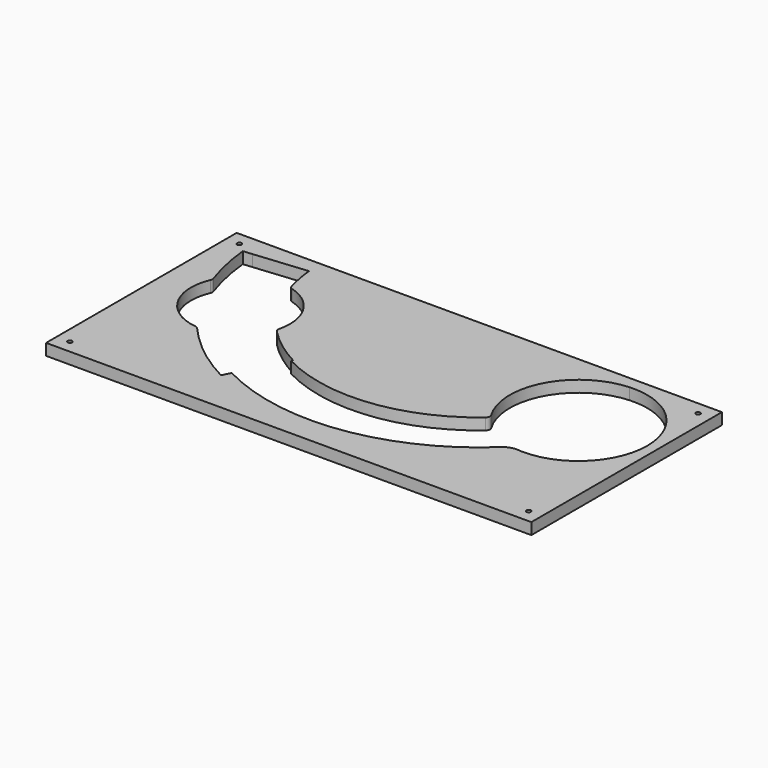
from build123d import *

# Parameters (mm, degrees)
F0_W     = 550
F0_H     = 270
F1_DEPTH = 13
F2_R     = 2.5
F3_DEPTH = 25
F4_R     = 5
F5_R     = 20


with BuildPart() as f1:
    # F0 (on Top) → F1 (new body)
    with BuildSketch(Plane.XY):
        with Locations((275, -135)):
            Rectangle(F0_W, F0_H)
    extrude(amount=-F1_DEPTH)

    # F2 (on face) → F3 (cut)
    with BuildSketch(Plane.XY):
        with BuildLine():
            ThreePointArc((102.8172889589, -52.4701250099), (119.1726628165, -90.0990620723), (143.6244940218, -123.0466433063))
            ThreePointArc((143.6244940218, -123.0466433063), (145.375436454, -115.11981647), (145.9631920321, -107.023216784))
            ThreePointArc((145.9631920321, -107.023216784), (133.8730301026, -72.2467564476), (102.8172889589, -52.4701250099))
        make_face()
        with BuildLine():
            ThreePointArc((46.4524007703, -71.5977994519), (67.6630708031, -119.8818075906), (98.9269281749, -162.353082441))
            ThreePointArc((98.9269281749, -162.353082441), (126.0574308053, -149.8675419291), (142.9268949098, -125.2225814773))
            ThreePointArc((142.9268949098, -125.2225814773), (117.4412479589, -91.100162762), (100.5834584289, -51.9891337337))
            ThreePointArc((100.5834584289, -51.9891337337), (70.8084957225, -54.3138897804), (46.4524007703, -71.5977994519))
        make_face()
        with BuildLine():
            ThreePointArc((36.6062109858, -22.9924196081), (40.2678425285, -47.5506492992), (46.4524007703, -71.5977994519))
            ThreePointArc((46.4524007703, -71.5977994519), (70.8084957225, -54.3138897804), (100.5834584289, -51.9891337337))
            ThreePointArc((100.5834584289, -51.9891337337), (96.3763447636, -34.89397928), (93.8406279725, -17.4723188671))
            Line((93.8406279725, -17.4723188671), (36.6062109858, -22.9924196081))
        make_face()
        with BuildLine():
            ThreePointArc((26.1547087534, -24.0004380043), (30.8880481953, -53.9384370008), (39.2095922874, -83.0835942334))
            ThreePointArc((39.2095922874, -83.0835942334), (42.4819606163, -77.1205988593), (46.4524007703, -71.5977994519))
            ThreePointArc((46.4524007703, -71.5977994519), (40.2678425285, -47.5506492992), (36.6062109858, -22.9924196081))
            Line((36.6062109858, -22.9924196081), (26.1547087534, -24.0004380043))
        make_face()
        with BuildLine():
            ThreePointArc((39.2095922874, -83.0835942334), (58.5731428007, -125.1375862115), (85.359218008, -162.8998889056))
            ThreePointArc((85.359218008, -162.8998889056), (92.159689712, -163.0387878421), (98.9269281749, -162.353082441))
            ThreePointArc((98.9269281749, -162.353082441), (67.6630708031, -119.8818075906), (46.4524007703, -71.5977994519))
            ThreePointArc((46.4524007703, -71.5977994519), (42.4819606163, -77.1205988593), (39.2095922874, -83.0835942334))
        make_face()
        with BuildLine():
            ThreePointArc((39.2095922874, -83.0835942334), (41.3696850637, -135.0845918815), (85.359218008, -162.8998889056))
            ThreePointArc((85.359218008, -162.8998889056), (58.5731428007, -125.1375862115), (39.2095922874, -83.0835942334))
        make_face()
        with BuildLine():
            ThreePointArc((98.9269281749, -162.353082441), (129.5126452175, -190.2463655327), (164.4445024089, -212.4564236553))
            Line((164.4445024089, -212.4564236553), (190.9870540226, -161.4491403142))
            ThreePointArc((190.9870540226, -161.4491403142), (165.4491613095, -145.3362093293), (142.9268949098, -125.2225814773))
            ThreePointArc((142.9268949098, -125.2225814773), (126.0574308053, -149.8675419291), (98.9269281749, -162.353082441))
        make_face()
        with BuildLine():
            ThreePointArc((85.359218008, -162.8998889056), (119.6639725539, -195.884452107), (159.5976016794, -221.7707971349))
            Line((159.5976016794, -221.7707971349), (164.4445024089, -212.4564236553))
            ThreePointArc((164.4445024089, -212.4564236553), (129.5126452175, -190.2463655327), (98.9269281749, -162.353082441))
            ThreePointArc((98.9269281749, -162.353082441), (92.159689712, -163.0387878421), (85.359218008, -162.8998889056))
        make_face()
        with BuildLine():
            ThreePointArc((142.9268949098, -125.2225814773), (165.4491613095, -145.3362093293), (190.9870540226, -161.4491403142))
            Line((190.9870540226, -161.4491403142), (191.9102732092, -159.6749739371))
            ThreePointArc((191.9102732092, -159.6749739371), (166.2146946142, -143.4076613439), (143.6244940218, -123.0466433063))
            ThreePointArc((143.6244940218, -123.0466433063), (143.2867819227, -124.1381669965), (142.9268949098, -125.2225814773))
        make_face()
        with BuildLine():
            Line((190.9870540226, -161.4491403142), (164.4445024089, -212.4564236553))
            ThreePointArc((164.4445024089, -212.4564236553), (312.3186805101, -236.5746522453), (445.5878496959, -168.1072144083))
            ThreePointArc((445.5878496959, -168.1072144083), (417.7995521532, -156.6837386519), (396.3969974723, -135.5978207964))
            ThreePointArc((396.3969974723, -135.5978207964), (297.7258554679, -180.5755672655), (190.9870540226, -161.4491403142))
        make_face()
        with BuildLine():
            ThreePointArc((396.3969974723, -135.5978207964), (417.7995521532, -156.6837386519), (445.5878496959, -168.1072144083))
            ThreePointArc((445.5878496959, -168.1072144083), (489.778644371, -105.9735057557), (512.2017629268, -33.0994511193))
            ThreePointArc((512.2017629268, -33.0994511193), (486.2288437534, -17.9967113583), (456.4729635167, -13.8406471114))
            ThreePointArc((456.4729635167, -13.8406471114), (438.2138341358, -80.5310148123), (396.3969974723, -135.5978207964))
        make_face()
        with BuildLine():
            ThreePointArc((395.2793152892, -133.9137271289), (395.8326968589, -134.7593972826), (396.3969974723, -135.5978207964))
            ThreePointArc((396.3969974723, -135.5978207964), (438.2138341358, -80.5310148123), (456.4729635167, -13.8406471114))
            ThreePointArc((456.4729635167, -13.8406471114), (391.3304963156, -56.2714595868), (395.2793152892, -133.9137271289))
        make_face()
        with BuildLine():
            ThreePointArc((445.5878496959, -168.1072144083), (452.1119253863, -169.1179747106), (458.6981361528, -169.5729777234))
            ThreePointArc((458.6981361528, -169.5729777234), (515.1450884683, -147.5010120731), (538.711061865, -91.6612861494))
            ThreePointArc((538.711061865, -91.6612861494), (531.7751165183, -59.5200686387), (512.2017629268, -33.0994511193))
            ThreePointArc((512.2017629268, -33.0994511193), (489.778644371, -105.9735057557), (445.5878496959, -168.1072144083))
        make_face()
        with BuildLine():
            ThreePointArc((17.5, -255), (13.232233047, -253.232233047), (15, -257.5))
            ThreePointArc((15, -257.5), (16.767766953, -256.767766953), (17.5, -255))
        make_face()
        with Locations((15, -15)):
            Circle(F2_R)
        with BuildLine():
            ThreePointArc((537.5, -15), (536.767766953, -13.232233047), (535, -12.5))
            ThreePointArc((535, -12.5), (533.232233047, -16.767766953), (537.5, -15))
        make_face()
        with Locations((535, -255)):
            Circle(F2_R)
        with BuildLine():
            ThreePointArc((100.5834584289, -51.9891337337), (117.4412479589, -91.100162762), (142.9268949098, -125.2225814773))
            ThreePointArc((142.9268949098, -125.2225814773), (143.2867819227, -124.1381669965), (143.6244940218, -123.0466433063))
            ThreePointArc((143.6244940218, -123.0466433063), (119.1726628165, -90.0990620723), (102.8172889589, -52.4701250099))
            ThreePointArc((102.8172889589, -52.4701250099), (101.702824577, -52.2182469254), (100.5834584289, -51.9891337337))
        make_face()
        with BuildLine():
            ThreePointArc((93.8406279725, -17.4723188671), (96.3763447636, -34.89397928), (100.5834584289, -51.9891337337))
            ThreePointArc((100.5834584289, -51.9891337337), (101.702824577, -52.2182469254), (102.8172889589, -52.4701250099))
            ThreePointArc((102.8172889589, -52.4701250099), (98.4454239564, -35.0497029669), (95.8313903025, -17.2803153631))
            Line((95.8313903025, -17.2803153631), (93.8406279725, -17.4723188671))
        make_face()
    extrude(amount=-F3_DEPTH, mode=Mode.SUBTRACT)

    # F4
    f4_edges = [f1.edges().sort_by_distance(p)[0] for p in [
        (102.817289, -52.470125, -6.5),
        (143.624494, -123.046643, -6.5),
        (39.209592, -83.083594, -6.5),
        (85.359218, -162.899889, -6.5),
        (396.396997, -135.597821, -6.5),
    ]]
    fillet(f4_edges, radius=F4_R)

    # F5
    f5_edges = [f1.edges().sort_by_distance(p)[0] for p in [
        (445.58785, -168.107214, -6.5),
    ]]
    fillet(f5_edges, radius=F5_R)


solid = f1.part
